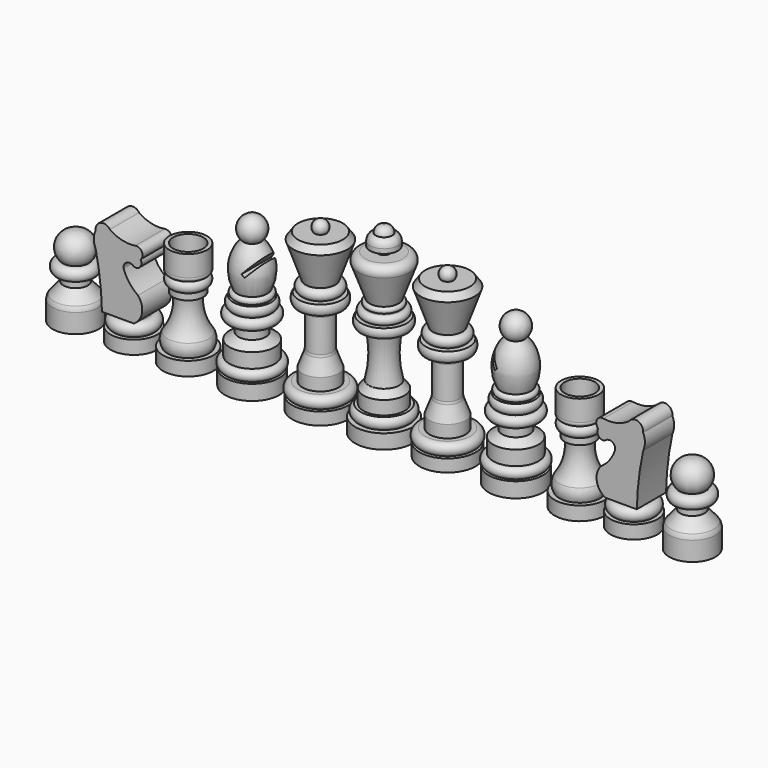
from build123d import *

# Parameters (mm, degrees)
F7_DEPTH = 12.7
F9_DEPTH = 190.5
F12_R    = 5.08
F12_2_R  = 5.08
F13_SIZE = 5.08
F14_SIZE = 5.08
F15_R    = 5.08
F16_R    = 5.08
F17_R    = 5.08


# Not quite as in the source:
# - a fillet or chamfer that OpenCascade refuses, or shapes differently, is made with other operations: its cross-section is extruded or revolved along the edge and cut away or added


with BuildPart() as f1:
    # F0 (on Front) → F1 (revolve)
    with BuildSketch(Plane.XZ):
        with BuildLine():
            Line((0, 90.6244069338), (0, -36.8451848626))
            Line((0, -36.8451848626), (20.1566442847, -36.8451848626))
            Line((20.1566442847, -36.8451848626), (20.1566442847, -26.7907716334))
            Line((20.1566442847, -26.7907716334), (16.2895619869, -26.7907716334))
            ThreePointArc((16.2895619869, -26.7907716334), (18.8838168485, -22.8463476524), (16.2895619869, -18.9019236714))
            Line((16.2895619869, -18.9019236714), (14.2786791548, -18.9019236714))
            Line((14.2786791548, -18.9019236714), (14.2786791548, -9.4662429765))
            Line((14.2786791548, -9.4662429765), (10.5662811548, -4.5163775794))
            ThreePointArc((10.5662811548, -4.5163775794), (8.4921483503, 12.189417379), (10.5662811548, 28.8952123374))
            Line((10.5662811548, 28.8952123374), (15.8255118877, 28.8952123374))
            ThreePointArc((15.8255118877, 28.8952123374), (16.9088707338, 32.0662213489), (15.8255118877, 35.2372303605))
            Line((15.8255118877, 35.2372303605), (11.8037471548, 35.2372303605))
            ThreePointArc((11.8037471548, 35.2372303605), (14.8974126205, 38.3308958262), (11.8037471548, 41.4245612919))
            Line((11.8037471548, 41.4245612919), (10.1022301242, 41.4245612919))
            ThreePointArc((10.1022301242, 41.4245612919), (12.1131138876, 43.4354450554), (10.1022301242, 45.4463288188))
            Line((10.1022301242, 45.4463288188), (20.50008066, 73.9273950458))
            Line((20.50008066, 73.9273950458), (4.0486049838, 73.9273950458))
            Line((4.0486049838, 73.9273950458), (4.0486049838, 77.6105523109))
            Line((4.0486049838, 77.6105523109), (9.6961269155, 77.6105523109))
            Line((9.6961269155, 77.6105523109), (9.6961269155, 85.7135280967))
            Line((9.6961269155, 85.7135280967), (5.767414812, 85.7135280967))
            Line((5.767414812, 85.7135280967), (5.767414812, 90.6244069338))
            Line((5.767414812, 90.6244069338), (0, 90.6244069338))
        make_face()
    revolve(axis=Axis((0, 0, 26.8896110356), (0, 0, -1)))

    # F11: fillet of radius 5.08 on 2 edges, made by hand

    # F11_s1 → F11_t2 (revolve, cut)
    with BuildSketch(Plane.XZ):
        with BuildLine():
            ThreePointArc((9.6961269155, 80.7657067398), (8.59450237, 83.9246509848), (5.767414812, 85.7135280967))
            Line((5.767414812, 85.7135280967), (9.6961269155, 85.7135280967))
            Line((9.6961269155, 85.7135280967), (9.6961269155, 80.7657067398))
        make_face()
    revolve(axis=Axis((0, 0, 85.7135280967), (0, 0, -1)), mode=Mode.SUBTRACT)

    # F11_s3 → F11_t4 (revolve, cut)
    with BuildSketch(Plane.XZ):
        with BuildLine():
            ThreePointArc((5.767414812, 85.7135280967), (4.2220337206, 89.1958132045), (0.6902307468, 90.6244069338))
            Line((0.6902307468, 90.6244069338), (5.767414812, 90.6244069338))
            Line((5.767414812, 90.6244069338), (5.767414812, 85.7135280967))
        make_face()
    revolve(axis=Axis((0, 0, 90.6244069338), (0, 0, -1)), mode=Mode.SUBTRACT)

    # F15
    f15_edges = [f1.edges().sort_by_distance(p)[0] for p in [
        (-20.500081, 0, 73.927395),
    ]]
    fillet(f15_edges, radius=F15_R)


with BuildPart() as f2:
    # F0 (on Front) → F2 (revolve)
    with BuildSketch(Plane.XZ):
        with BuildLine():
            Line((-91.6927829385, 67.1136900783), (-91.6927829385, -37.4382734299))
            Line((-91.6927829385, -37.4382734299), (-72.6825594902, -37.4382734299))
            Line((-72.6825594902, -37.4382734299), (-72.6825594902, -26.9498731941))
            Line((-72.6825594902, -26.9498731941), (-75.9601816535, -26.9498731941))
            ThreePointArc((-75.9601816535, -26.9498731941), (-72.1909133717, -23.1806049123), (-75.9601816535, -19.4113366306))
            Line((-75.9601816535, -19.4113366306), (-75.9601816535, -9.2506995425))
            Line((-75.9601816535, -9.2506995425), (-82.1876674891, -4.9897874705))
            Line((-82.1876674891, -4.9897874705), (-82.1876674891, 2.8765120078))
            Line((-82.1876674891, 2.8765120078), (-78.5822793841, 2.8765120078))
            ThreePointArc((-78.5822793841, 2.8765120078), (-74.8130112188, 6.6457801731), (-78.5822793841, 10.4150483385))
            ThreePointArc((-78.5822793841, 10.4150483385), (-76.8449475986, 13.8565548696), (-78.5822793841, 17.2980614007))
            Line((-78.5822793841, 17.2980614007), (-81.1222793841, 17.2980614007))
            ThreePointArc((-81.1222793841, 17.2980614007), (-78.8447114015, 19.5756293833), (-81.1222793841, 21.853197366))
            ThreePointArc((-81.1222793841, 21.853197366), (-78.7317250175, 37.598761469), (-85.6791585684, 51.9295223057))
            ThreePointArc((-85.6791585684, 51.9295223057), (-83.4614511239, 61.5907547312), (-91.6927829385, 67.1136900783))
        make_face()
    revolve(axis=Axis((-91.6927829385, 0, 14.8377083242), (0, 0, -1)))

    # F6 (on Front) → F9 (cut, symmetric)
    with BuildSketch(Plane.XZ):
        Polygon((-88.8920841115, 36.408969577), (-86.9335755706, 34.658677876), (-75.517475605, 47.4328510463), (-77.4759841459, 49.1831427473), align=None)
    extrude(amount=F9_DEPTH, both=True, mode=Mode.SUBTRACT)


with BuildPart() as f3:
    # F0 (on Front) → F3 (revolve)
    with BuildSketch(Plane.XZ):
        with BuildLine():
            Line((-136.1957192421, 23.021209985), (-136.1957192421, -37.7154462039))
            Line((-136.1957192421, -37.7154462039), (-118.6755225062, -37.7154462039))
            Line((-118.6755225062, -37.7154462039), (-118.6755225062, -28.0793458223))
            Line((-118.6755225062, -28.0793458223), (-121.8875572085, -28.0793458223))
            ThreePointArc((-121.8875572085, -28.0793458223), (-120.6610963132, -23.5532959923), (-121.8875572085, -19.0272461623))
            ThreePointArc((-121.8875572085, -19.0272461623), (-127.183201187, -7.4815513153), (-127.7276277542, 5.2090166137))
            Line((-127.7276277542, 5.2090166137), (-125.6835907698, 5.2090166137))
            Line((-125.6835907698, 5.2090166137), (-125.6835907698, 9.589063935))
            ThreePointArc((-125.6835907698, 9.589063935), (-123.0764808508, 13.3851054125), (-125.6835907698, 17.1811468899))
            ThreePointArc((-125.6835907698, 17.1811468899), (-123.5036213666, 18.0758055538), (-123.0764808508, 20.3931815922))
            Line((-123.0764808508, 20.3931815922), (-123.0764808508, 34.99333933))
            Line((-123.0764808508, 34.99333933), (-125.6835907698, 34.99333933))
            Line((-125.6835907698, 34.99333933), (-125.6835907698, 23.021209985))
            Line((-125.6835907698, 23.021209985), (-136.1957192421, 23.021209985))
        make_face()
    revolve(axis=Axis((-136.1957192421, 0, -7.3471181095), (0, 0, -1)))


with BuildPart() as f4:
    # F0 (on Front) → F4 (revolve)
    with BuildSketch(Plane.XZ):
        with BuildLine():
            Line((-173.8641262054, -19.5217264038), (-173.8641262054, -37.3339169812))
            Line((-173.8641262054, -37.3339169812), (-157.511934638, -37.3339169812))
            Line((-157.511934638, -37.3339169812), (-157.511934638, -27.9898197544))
            Line((-157.511934638, -27.9898197544), (-160.4319661856, -27.9898197544))
            ThreePointArc((-160.4319661856, -27.9898197544), (-158.5045092712, -22.2332221282), (-163.9360189438, -19.5217264038))
            Line((-163.9360189438, -19.5217264038), (-173.8641262054, -19.5217264038))
        make_face()
    revolve(axis=Axis((-173.8641262054, 0, -28.4278216925), (0, 0, -1)))


with BuildPart() as f5:
    # F0 (on Front) → F5 (revolve)
    with BuildSketch(Plane.XZ):
        with BuildLine():
            Line((-214.4525647163, 17.4731574953), (-214.4525647163, -38.0074456334))
            Line((-214.4525647163, -38.0074456334), (-198.3923912048, -38.0074456334))
            Line((-198.3923912048, -38.0074456334), (-198.3923912048, -22.8232797235))
            Line((-198.3923912048, -22.8232797235), (-205.9844881296, -13.7711809948))
            Line((-205.9844881296, -13.7711809948), (-205.9844881296, -7.6391142793))
            Line((-205.9844881296, -7.6391142793), (-201.6044408083, -7.6391142793))
            ThreePointArc((-201.6044408083, -7.6391142793), (-200.871972485, -2.5124192135), (-205.4004669189, 0))
            ThreePointArc((-205.4004669189, 0), (-203.7502551855, 11.9362360093), (-214.4525647163, 17.4731574953))
        make_face()
    revolve(axis=Axis((-214.4525647163, 0, -10.2671440691), (0, 0, -1)))


with BuildPart() as f7:
    # F6 (on Front) → F7 (new body, symmetric)
    with BuildSketch(Plane.XZ):
        with BuildLine():
            ThreePointArc((-190.4150545597, 19.122518599), (-187.2931587384, 0.5872536702), (-185.9959065914, -18.1642640382))
            Line((-185.9959065914, -18.1642640382), (-163.9002263546, -18.1642640382))
            ThreePointArc((-163.9002263546, -18.1642640382), (-158.122108873, -9.7803789383), (-160.9541326761, 0))
            ThreePointArc((-160.9541326761, 0), (-167.0109154815, 5.8124570625), (-170.8971858025, 13.2533023134))
            ThreePointArc((-170.8971858025, 13.2533023134), (-168.704403711, 17.625731253), (-163.9002263546, 16.7057812214))
            ThreePointArc((-163.9002263546, 16.7057812214), (-159.4143131156, 17.9338152242), (-159.1128110886, 22.5749984384))
            ThreePointArc((-159.1128110886, 22.5749984384), (-158.2079342422, 27.5949767588), (-162.7954244614, 29.8252049834))
            ThreePointArc((-162.7954244614, 29.8252049834), (-172.0342004876, 30.1879269413), (-180.4719865322, 33.968180418))
            ThreePointArc((-180.4719865322, 33.968180418), (-186.9386070045, 35.9836973027), (-190.4150545597, 30.1704537123))
            ThreePointArc((-190.4150545597, 30.1704537123), (-191.6338166601, 24.6464861557), (-190.4150545597, 19.122518599))
        make_face()
    extrude(amount=F7_DEPTH, both=True)


with BuildPart() as f8:
    # F6 (on Front) → F8 (revolve)
    with BuildSketch(Plane.XZ):
        with BuildLine():
            ThreePointArc((-40.1643700898, 71.9454586506), (-39.8036635375, 77.0157852023), (-44.2152433097, 79.5409157872))
            Line((-44.2152433097, 79.5409157872), (-44.2152433097, -36.8076525629))
            Line((-44.2152433097, -36.8076525629), (-24.697387591, -36.8076525629))
            Line((-24.697387591, -36.8076525629), (-24.697387591, -28.1764548272))
            Line((-24.697387591, -28.1764548272), (-28.3800046891, -28.1764548272))
            ThreePointArc((-28.3800046891, -28.1764548272), (-24.0644048899, -23.860855028), (-28.3800046891, -19.5452552289))
            Line((-28.3800046891, -19.5452552289), (-31.6943563521, -19.5452552289))
            Line((-31.6943563521, -19.5452552289), (-31.6943563521, -10.9140556306))
            Line((-31.6943563521, -10.9140556306), (-35.7452332973, 0))
            Line((-35.7452332973, 0), (-35.7452332973, 23.6107409))
            ThreePointArc((-35.7452332973, 23.6107409), (-33.6215477296, 27.613361561), (-29.1165281087, 28.0989650637))
            ThreePointArc((-29.1165281087, 28.0989650637), (-28.0016383786, 31.5514458343), (-29.1165281087, 35.003926605))
            Line((-29.1165281087, 35.003926605), (-33.9047345445, 35.003926605))
            ThreePointArc((-33.9047345445, 35.003926605), (-30.1070078389, 38.8016533107), (-33.9047345445, 42.5993800163))
            Line((-33.9047345445, 42.5993800163), (-23.5926061869, 71.9454586506))
            Line((-23.5926061869, 71.9454586506), (-40.1643700898, 71.9454586506))
        make_face()
    revolve(axis=Axis((-44.2152433097, 0, 21.3666316122), (0, 0, -1)))


with BuildPart() as f10_1:
    # F10: instance of F7
    add(f7.part.mirror(Plane.YZ))


with BuildPart() as f10_2:
    # F10: instance of F3
    add(f3.part.mirror(Plane.YZ))


with BuildPart() as f10_3:
    # F10: instance of F5
    add(f5.part.mirror(Plane.YZ))

    # F12#2
    f12_2_edges = [f10_3.edges().sort_by_distance(p)[0] for p in [
        (230.512738, 0, -22.82328),
    ]]
    fillet(f12_2_edges, radius=F12_2_R)


with BuildPart() as f10_4:
    # F10: instance of F4
    add(f4.part.mirror(Plane.YZ))


with BuildPart() as f10_5:
    # F10: instance of F8
    add(f8.part.mirror(Plane.YZ))

    # F13
    f13_edges = [f10_5.edges().sort_by_distance(p)[0] for p in [
        (64.83788, 0, 71.945459),
    ]]
    chamfer(f13_edges, length=F13_SIZE)

    # F17
    f17_edges = [f10_5.edges().sort_by_distance(p)[0] for p in [
        (52.685253, 0, 0),
    ]]
    fillet(f17_edges, radius=F17_R)


with BuildPart() as f10_6:
    # F10: instance of F2
    add(f2.part.mirror(Plane.YZ))


with BuildPart() as f5_1:
    add(f5.part)

    # F12
    f12_edges = [f5_1.edges().sort_by_distance(p)[0] for p in [
        (-230.512738, 0, -22.82328),
    ]]
    fillet(f12_edges, radius=F12_R)


with BuildPart() as f8_1:
    add(f8.part)

    # F14
    f14_edges = [f8_1.edges().sort_by_distance(p)[0] for p in [
        (-64.83788, 0, 71.945459),
    ]]
    chamfer(f14_edges, length=F14_SIZE)

    # F16
    f16_edges = [f8_1.edges().sort_by_distance(p)[0] for p in [
        (-52.685253, 0, 0),
    ]]
    fillet(f16_edges, radius=F16_R)


solid = Compound([f1.part, f2.part, f3.part, f4.part, f7.part, f10_1.part, f10_2.part, f10_3.part, f10_4.part, f10_5.part, f10_6.part, f5_1.part, f8_1.part])
